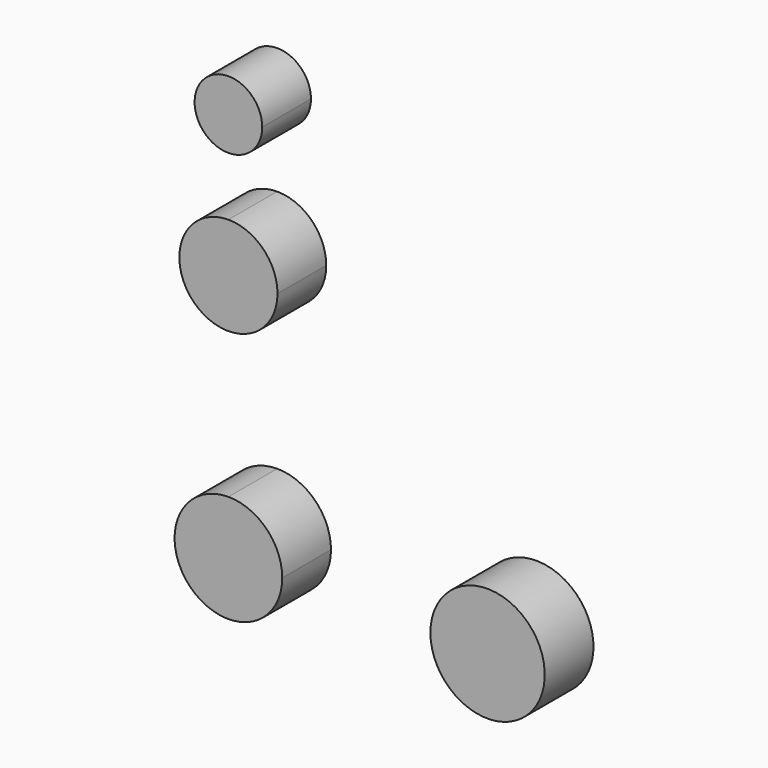
from build123d import *

# Parameters (mm, degrees)
F3_DEPTH = 25.4


# Not quite as in the source:
# - the program builds the solid bodies; features that only make, move or delete a surface that nothing else refers to are left out


with BuildPart() as f3:
    # F0 (on Front) → F3 (new body)
    with BuildSketch(Plane.XZ):
        with BuildLine():
            Line((22.4317827104, 0), (0, 0))
            Line((0, 0), (0, 22.4317827104))
            ThreePointArc((0, 22.4317827104), (-15.8616656686, -15.8616656686), (22.4317827104, 0))
        make_face()
        with BuildLine():
            Line((0, 22.4317827104), (0, 0))
            Line((0, 0), (22.4317827104, 0))
            ThreePointArc((22.4317827104, 0), (15.8616656686, 15.8616656686), (0, 22.4317827104))
        make_face()
    extrude(amount=F3_DEPTH)


with BuildPart() as f3b:
    # F0 (on Front) → F3, piece 2 (new body)
    with BuildSketch(Plane.XZ):
        with BuildLine():
            ThreePointArc((14.0866758828, 162.6749411225), (-9.9607840411, 172.6357251636), (0, 148.5882652397))
            ThreePointArc((0, 148.5882652397), (9.9607840411, 152.7141570814), (14.0866758828, 162.6749411225))
        make_face()
    extrude(amount=F3_DEPTH)


with BuildPart() as f3c:
    # F0 (on Front) → F3, piece 3 (new body)
    with BuildSketch(Plane.XZ):
        with BuildLine():
            ThreePointArc((0, 124.1158500545), (-20.4522788755, 103.6635711789), (0, 83.2112923034))
            Line((0, 83.2112923034), (0, 124.1158500545))
        make_face()
        with BuildLine():
            Line((0, 124.1158500545), (0, 83.2112923034))
            ThreePointArc((0, 83.2112923034), (14.4619450836, 89.2016260953), (20.4522788755, 103.6635711789))
            ThreePointArc((20.4522788755, 103.6635711789), (14.4619450836, 118.1255162625), (0, 124.1158500545))
        make_face()
    extrude(amount=F3_DEPTH)


with BuildPart() as f3d:
    # F0 (on Front) → F3, piece 4 (new body)
    with BuildSketch(Plane.XZ):
        with BuildLine():
            ThreePointArc((131.8241035994, 0), (107.9986616969, 23.8254419025), (84.1732197944, 0))
            ThreePointArc((84.1732197944, 0), (107.9986616969, -23.8254419025), (131.8241035994, 0))
        make_face()
    extrude(amount=F3_DEPTH)


solid = Compound([f3.part, f3b.part, f3c.part, f3d.part])
